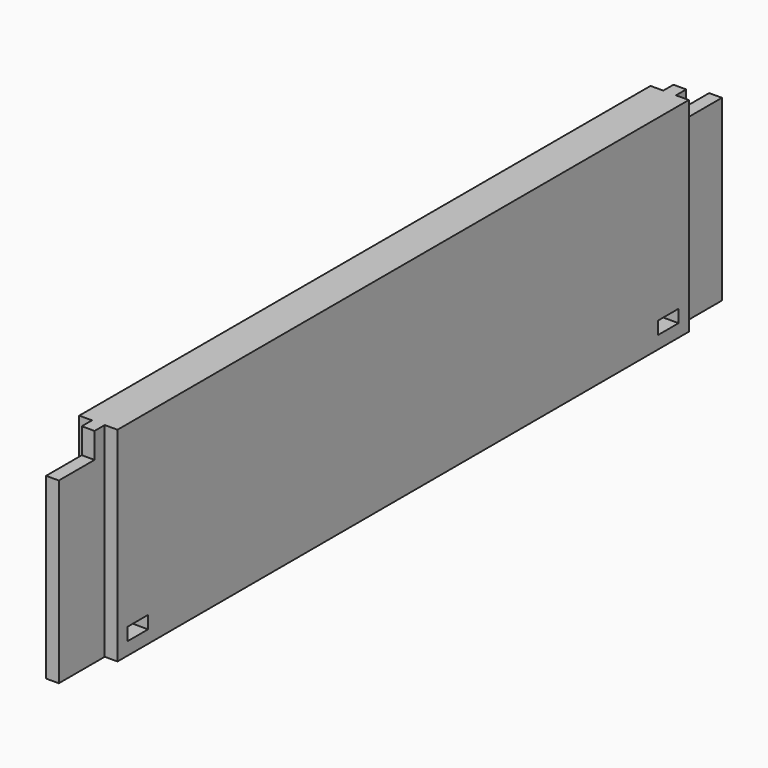
from build123d import *

# Parameters (mm, degrees)
F0_W     = 355.6
F0_H     = 101.6
F1_DEPTH = 9.525
F2_DEPTH = 3.175
F3_W     = 12.7
F3_H     = 6.35
F4_DEPTH = 12.7


# Not quite as in the source:
# - a feature names something its author has since deleted; it is built from what else it names


with BuildPart() as f1:
    # F0 (on Right) → F1 (new body, symmetric)
    with BuildSketch(Plane.YZ):
        with Locations((0, -50.8)):
            Rectangle(F0_W, F0_H)
    extrude(amount=F1_DEPTH, both=True)

    # F0 (on Right) → F2 (join, symmetric)
    with BuildSketch(Plane.YZ):
        Polygon((-177.8, -101.6), (-177.8, 0), (-184.15, 0), (-184.15, -12.7), (-206.375, -12.7), (-206.375, -101.6), align=None)
        Polygon((184.15, 0), (177.8, 0), (177.8, -101.6), (206.375, -101.6), (206.375, -12.7), (184.15, -12.7), align=None)
    extrude(amount=F2_DEPTH, both=True)

    # F3 (on face) → F4 (cut)
    with BuildSketch(Plane.YZ.offset(9.525)):
        with Locations((-165.1, -92.075)):
            Rectangle(F3_W, F3_H)
        with Locations((165.1, -92.075)):
            Rectangle(F3_W, F3_H)
    extrude(amount=-F4_DEPTH, mode=Mode.SUBTRACT)


solid = f1.part
